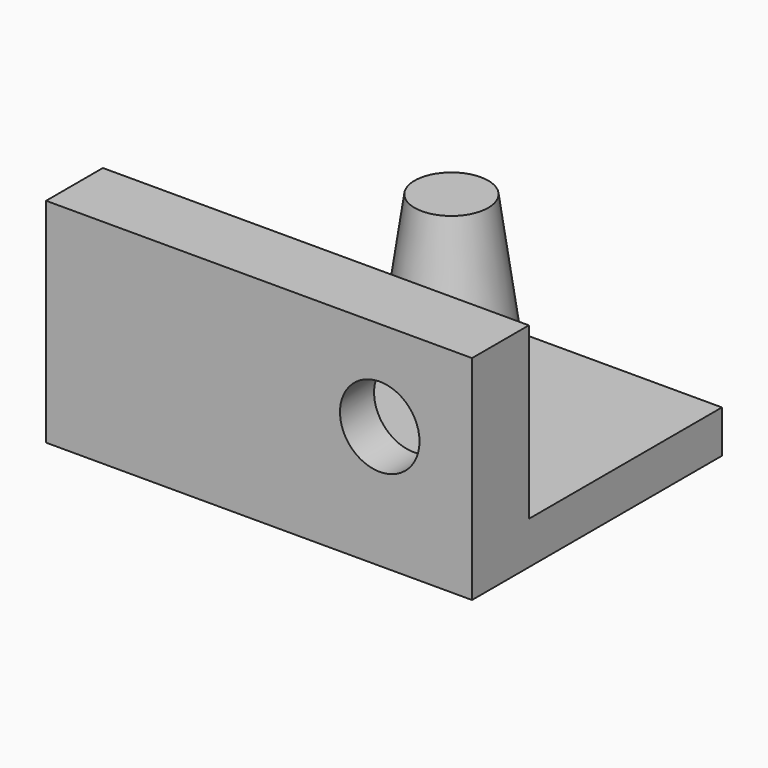
from build123d import *

# Parameters (mm, degrees)
F0_W           = 30
F0_H           = 22
F1_DEPTH       = 3
F2_W           = 30
F2_H           = 5
F2_R           = 4
F3_DEPTH       = 10
F3_TAPER       = 8
F4_DEPTH       = 12
F6_D           = 5.6
F6_DEPTH       = 15
F6_CBORE_D     = 10
F6_CBORE_DEPTH = 2
F6_TIP         = 1.6824097333


with BuildPart() as f1:
    # F0 (on Top) → F1 (new body)
    with BuildSketch(Plane.XY):
        with Locations((0.4801530018, 11)):
            Rectangle(F0_W, F0_H)
    extrude(amount=F1_DEPTH)

    # F2 (on face) → F3 (join)
    with BuildSketch(Plane.XY.offset(3)):
        with Locations((0.4801530018, 2.5)):
            Rectangle(F2_W, F2_H)
        with Locations((0, 17.5365079194)):
            Circle(F2_R)
    extrude(amount=F3_DEPTH, taper=F3_TAPER)

    # F2 (on face) → F4 (join)
    with BuildSketch(Plane.XY.offset(3)):
        with Locations((0.4801530018, 2.5)):
            Rectangle(F2_W, F2_H)
    extrude(amount=F4_DEPTH)

    # F6
    with Locations(Plane(origin=(0, 5, 0), x_dir=(-1, 0, 0), z_dir=(0, 1, 0))):
        with Locations((-8.9809922501, 8.6309639737)):
            CounterBoreHole(F6_D / 2, F6_CBORE_D / 2, F6_CBORE_DEPTH, depth=F6_DEPTH)
            with Locations((0, 0, -(F6_DEPTH + F6_TIP / 2))):  # 118° drill point
                Cone(0, F6_D / 2, F6_TIP, mode=Mode.SUBTRACT)


solid = f1.part
